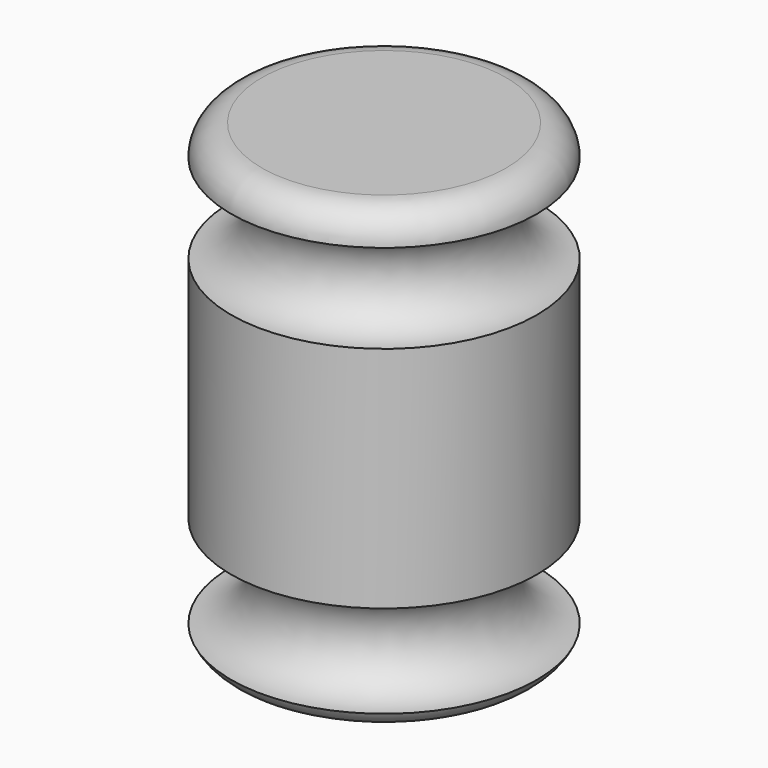
from build123d import *


# Not quite as in the source:
# - a fillet or chamfer that OpenCascade refuses, or shapes differently, is made with other operations: its cross-section is extruded or revolved along the edge and cut away or added


with BuildPart() as f1:
    # F0 (on Front) → F1 (revolve)
    with BuildSketch(Plane.XZ):
        with BuildLine():
            Line((-28.9062019438, 2.8610236477), (-3.5062019438, 2.8610236477))
            Line((-3.5062019438, 2.8610236477), (-3.5062019438, 5.8150213674))
            ThreePointArc((-3.5062019438, 5.8150213674), (-11.2070506632, 13.5158700868), (-3.5062019438, 21.2167188063))
            Line((-3.5062019438, 21.2167188063), (-3.5062019438, 59.2063053419))
            ThreePointArc((-3.5062019438, 59.2063053419), (-10.8926867883, 66.5927901864), (-3.5062019438, 73.9792750309))
            Line((-3.5062019438, 73.9792750309), (-3.5062019438, 79.0610236477))
            Line((-3.5062019438, 79.0610236477), (-28.9062019438, 79.0610236477))
            Line((-28.9062019438, 79.0610236477), (-28.9062019438, 2.8610236477))
        make_face()
    revolve(axis=Axis((-28.9062019438, 0, 40.9610236477), (0, 0, 1)))

    # F2: fillet of radius 5.08 on 2 edges, made by hand

    # F2_s1 → F2_t2 (revolve, cut)
    with BuildSketch(Plane.XZ):
        with BuildLine():
            ThreePointArc((-3.5062019438, 73.9810236477), (-4.9940994953, 77.5731260961), (-8.5862019438, 79.0610236477))
            Line((-8.5862019438, 79.0610236477), (-8.5862019438, 79.1626236477))
            Line((-8.5862019438, 79.1626236477), (-3.4046019438, 79.1626236477))
            Line((-3.4046019438, 79.1626236477), (-3.4046019438, 73.9810236477))
            Line((-3.4046019438, 73.9810236477), (-3.5062019438, 73.9810236477))
        make_face()
    revolve(axis=Axis((-28.9062019438, 0, 79.0610236477), (0, 0, 1)), mode=Mode.SUBTRACT)

    # F2_s3 → F2_t4 (revolve, cut)
    with BuildSketch(Plane.XZ):
        with BuildLine():
            ThreePointArc((-8.1199330049, 2.8610236477), (-5.3807444009, 3.6627943654), (-3.5062019438, 5.8150213674))
            Line((-3.5062019438, 5.8150213674), (-3.4139273225, 5.7725013218))
            ThreePointArc((-3.4139273225, 5.7725013218), (-3.4046019438, 4.3380225076), (-3.4046019438, 2.8610236477))
            Line((-3.4046019438, 2.8610236477), (-3.5062019438, 2.7594236477))
            Line((-3.5062019438, 2.7594236477), (-8.1199330049, 2.7594236477))
            Line((-8.1199330049, 2.7594236477), (-8.1199330049, 2.8610236477))
        make_face()
    revolve(axis=Axis((-28.9062019438, 0, 2.8610236477), (0, 0, 1)), mode=Mode.SUBTRACT)


solid = f1.part
